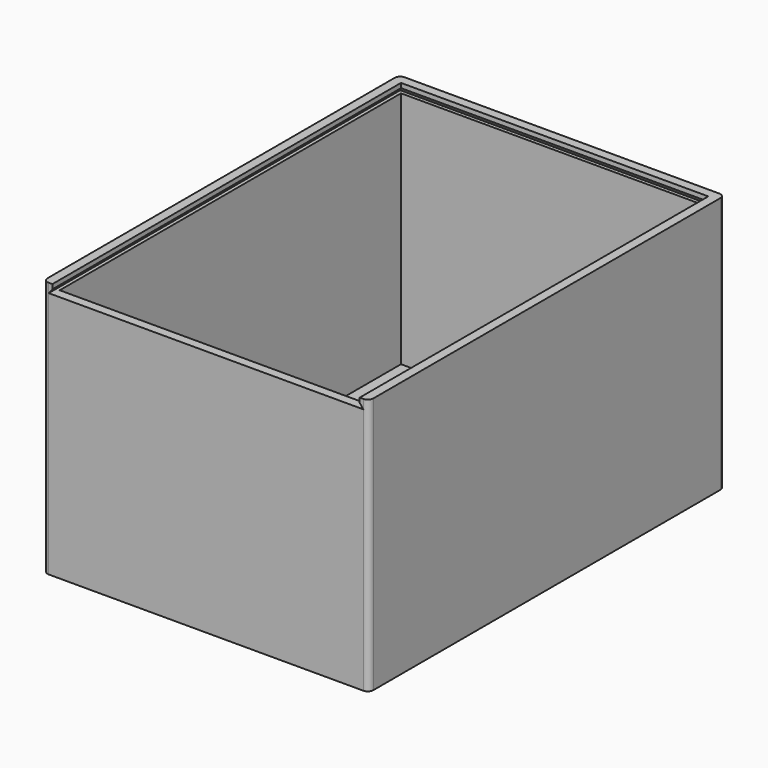
from build123d import *

# Parameters (mm, degrees)
F0_W     = 71
F0_H     = 54
F1_DEPTH = 97
F2_T     = -2
F4_DEPTH = 97
F6_DEPTH = 71
F7_R     = 1.19999


# Not quite as in the source:
# - a fillet or chamfer is up to 0.001 mm smaller than in the source, because OpenCascade refuses the exact size


with BuildPart() as f1:
    # F0 (on Front) → F1 (new body)
    with BuildSketch(Plane.XZ):
        with Locations((35.5, -27)):
            Rectangle(F0_W, F0_H)
    extrude(amount=-F1_DEPTH)

    # F2
    f2_openings = [f1.faces().sort_by_distance(p)[0] for p in [
        (35.5, 48.5, 0),
    ]]
    offset(amount=F2_T, openings=f2_openings)

    # F3 (on face) → F4 (join, through all)
    with BuildSketch(Plane.XZ):
        Polygon((0, 2), (0, 0), (1.2, 0), (2, 1), (2, 2), align=None)
        Polygon((69, 1), (69.8, 0), (71, 0), (71, 2), (69, 2), align=None)
    extrude(amount=-F4_DEPTH)

    # F5 (on face) → F6 (join, through all)
    with BuildSketch(Plane.YZ.offset(71)):
        Polygon((97, 0), (97, 2), (95, 2), (95, 1), (95.8, 0), align=None)
    extrude(amount=-F6_DEPTH)

    # F7 (radius 1.2 in the source; OpenCascade refuses exactly that, so slightly less here)
    f7_edges = [f1.edges().sort_by_distance(p)[0] for p in [
        (71, 0, -26),
        (71, 97, -26),
        (0, 0, -26),
        (0, 97, -26),
    ]]
    fillet(f7_edges, radius=F7_R)


solid = f1.part
